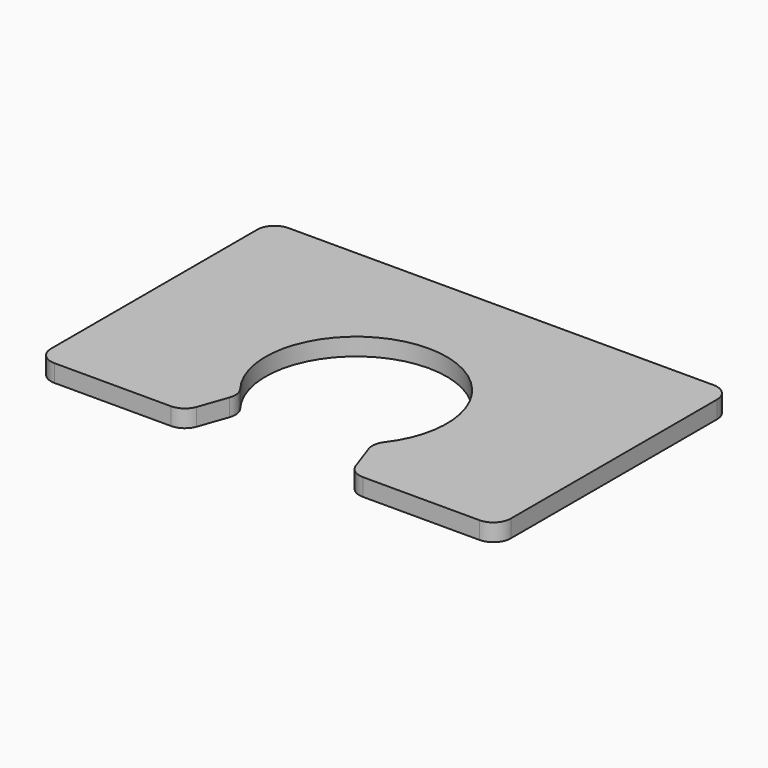
from build123d import *

# Parameters (mm, degrees)
F1_DEPTH    = 25
F2_T1_DEPTH = 150
F2_T3_DEPTH = 113.556925296
F2_T5_DEPTH = 96.327528549
F2_T7_DEPTH = 96.2047902339
F2_T9_DEPTH = 113.6738307778


# Not quite as in the source:
# - a fillet or chamfer that OpenCascade refuses, or shapes differently, is made with other operations: its cross-section is extruded or revolved along the edge and cut away or added


with BuildPart() as f1:
    # F0 (on Top) → F1 (new body)
    with BuildSketch(Plane.XY):
        with BuildLine():
            Line((330, -210), (330, 210))
            Line((330, 210), (-330, 210))
            Line((-330, 210), (-330, -210))
            Line((-330, -210), (-120, -210))
            Line((-120, -210), (-94.9556464673, -138.7567549117))
            ThreePointArc((-94.9556464673, -138.7567549117), (-47.6770453611, 70.9299598508), (130.0298179868, -50))
            ThreePointArc((130.0298179868, -50), (120.9675904588, -97.6870547372), (95.0443535327, -138.7256334719))
            Line((95.0443535327, -138.7256334719), (120, -210))
            Line((120, -210), (330, -210))
        make_face()
    extrude(amount=F1_DEPTH)

    # F2: fillet of radius 25 on 9 edges, made by hand

    # F2_s2 → F2_t1 (cut)
    with BuildSketch(Plane.XY.offset(-62.5)):
        with BuildLine():
            ThreePointArc((330, -185), (322.6776695297, -202.6776695297), (305, -210))
            Line((305, -210), (330, -210))
            Line((330, -210), (330, -185))
        make_face()
        with BuildLine():
            ThreePointArc((-330, -185), (-322.6776695297, -202.6776695297), (-305, -210))
            Line((-305, -210), (-330, -210))
            Line((-330, -210), (-330, -185))
        make_face()
        with BuildLine():
            ThreePointArc((330, 185), (322.6776695297, 202.6776695297), (305, 210))
            Line((305, 210), (330, 210))
            Line((330, 210), (330, 185))
        make_face()
        with BuildLine():
            ThreePointArc((-305, 210), (-322.6776695297, 202.6776695297), (-330, 185))
            Line((-330, 185), (-330, 210))
            Line((-330, 210), (-305, 210))
        make_face()
    extrude(amount=F2_T1_DEPTH, mode=Mode.SUBTRACT)

    # F2_s4 → F2_t3 (cut)
    with BuildSketch(Plane.XY.offset(-44.278462648)):
        with BuildLine():
            ThreePointArc((-137.7113850592, -210), (-123.2592934135, -205.3994374203), (-114.1262219297, -193.2909637652))
            Line((-114.1262219297, -193.2909637652), (-120, -210))
            Line((-120, -210), (-137.7113850592, -210))
        make_face()
    extrude(amount=F2_T3_DEPTH, mode=Mode.SUBTRACT)

    # F2_s6 → F2_t5 (cut)
    with BuildSketch(Plane.XY.offset(-35.6637642745)):
        with BuildLine():
            ThreePointArc((-99.6866381045, -152.2149260833), (-98.5772005252, -140.0282344234), (-103.3844432952, -128.7749361378))
            ThreePointArc((-103.3844432952, -128.7749361378), (-99.2955159897, -133.8717952023), (-94.9556464673, -138.7567549117))
            Line((-94.9556464673, -138.7567549117), (-99.6866381045, -152.2149260833))
        make_face()
    extrude(amount=F2_T5_DEPTH, mode=Mode.SUBTRACT)

    # F2_s8 → F2_t7 (cut)
    with BuildSketch(Plane.XY.offset(-35.6023951169)):
        with BuildLine():
            ThreePointArc((103.4562444176, -128.7589633994), (98.6534687448, -139.9957269325), (99.7504758881, -152.1665150823))
            Line((99.7504758881, -152.1665150823), (95.0443535327, -138.7256334719))
            ThreePointArc((95.0443535327, -138.7256334719), (99.3753638137, -133.8478534272), (103.4562444176, -128.7589633994))
        make_face()
    extrude(amount=F2_T7_DEPTH, mode=Mode.SUBTRACT)

    # F2_s10 → F2_t9 (cut)
    with BuildSketch(Plane.XY.offset(-44.3369153889)):
        with BuildLine():
            ThreePointArc((114.1393002355, -193.261597183), (123.2699801146, -205.3904380725), (137.7347661556, -210))
            Line((137.7347661556, -210), (120, -210))
            Line((120, -210), (114.1393002355, -193.261597183))
        make_face()
    extrude(amount=F2_T9_DEPTH, mode=Mode.SUBTRACT)


solid = f1.part
